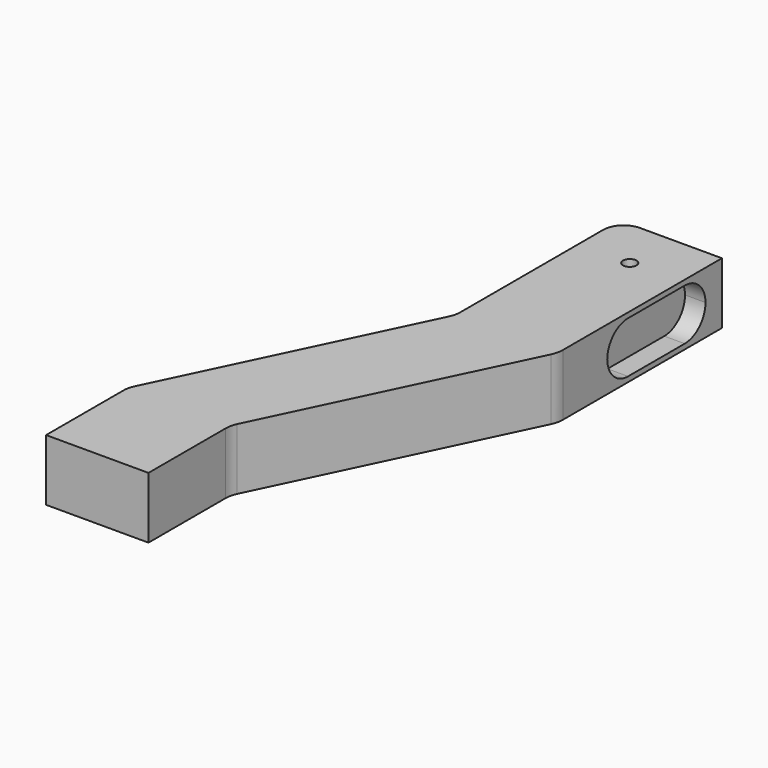
from build123d import *

# Parameters (mm, degrees)
F1_DEPTH    = 30
F2_W        = 60
F2_H        = 25
F3_DEPTH    = 10
F4_R        = 10
F5_R        = 3.2639
F6_DEPTH    = 30.001
F7_T1_DEPTH = 30
F7_T3_DEPTH = 10
F7_T5_DEPTH = 41.75
F7_T7_DEPTH = 44.4507439359


# Not quite as in the source:
# - a fillet or chamfer that OpenCascade refuses, or shapes differently, is made with other operations: its cross-section is extruded or revolved along the edge and cut away or added


with BuildPart() as f1:
    # F0 (on Top) → F1 (new body)
    with BuildSketch(Plane.XY):
        Polygon((-25, -100), (-25, -150), (25, -150), (25, -100), (85, 25), (85, 125), (35, 125), (35, 25), align=None)
    extrude(amount=F1_DEPTH)

    # F2 (on face) → F3 (cut)
    with BuildSketch(Plane.YZ.offset(85)):
        with Locations((85, 15)):
            Rectangle(F2_W, F2_H)
    extrude(amount=-F3_DEPTH, mode=Mode.SUBTRACT)

    # F4
    f4_edges = [f1.edges().sort_by_distance(p)[0] for p in [
        (35, 125, 15),
    ]]
    fillet(f4_edges, radius=F4_R)

    # F5 (on face) → F6 (cut, through all)
    with BuildSketch(Plane.XY.offset(30)):
        with Locations((60, 100)):
            Circle(F5_R)
    extrude(amount=-F6_DEPTH, mode=Mode.SUBTRACT)

    # F7: fillet of radius 12.7 on 8 edges, made by hand

    # F7_s2 → F7_t1 (join)
    with BuildSketch(Plane.XY):
        with BuildLine():
            ThreePointArc((26.2506571702, -97.3944642288), (25.3166108448, -100.0720513739), (25, -102.8901487872))
            Line((25, -102.8901487872), (25, -100))
            Line((25, -100), (26.2506571702, -97.3944642288))
        make_face()
        with BuildLine():
            ThreePointArc((35, 27.8901487872), (34.6833891552, 25.0720513739), (33.7493428298, 22.3944642288))
            Line((33.7493428298, 22.3944642288), (35, 25))
            Line((35, 25), (35, 27.8901487872))
        make_face()
    extrude(amount=F7_T1_DEPTH)

    # F7_s4 → F7_t3 (join)
    with BuildSketch(Plane.YZ.offset(75)):
        with BuildLine():
            ThreePointArc((102.3, 27.5), (111.2802561211, 23.7802561211), (115, 14.8))
            Line((115, 14.8), (115, 27.5))
            Line((115, 27.5), (102.3, 27.5))
        make_face()
        with BuildLine():
            ThreePointArc((115, 15.2), (111.2802561211, 6.2197438789), (102.3, 2.5))
            Line((102.3, 2.5), (115, 2.5))
            Line((115, 2.5), (115, 15.2))
        make_face()
    extrude(amount=F7_T3_DEPTH)

    # F7_s6 → F7_t5 (join)
    with BuildSketch(Plane.YZ.offset(43.25)):
        with BuildLine():
            ThreePointArc((67.7, 27.5), (58.7197438789, 23.7802561211), (55, 14.8))
            Line((55, 14.8), (55, 27.5))
            Line((55, 27.5), (67.7, 27.5))
        make_face()
        with BuildLine():
            ThreePointArc((67.7, 2.5), (58.7197438789, 6.2197438789), (55, 15.2))
            Line((55, 15.2), (55, 2.5))
            Line((55, 2.5), (67.7, 2.5))
        make_face()
    extrude(amount=F7_T5_DEPTH)

    # F7_s8 → F7_t7 (cut)
    with BuildSketch(Plane.XY.offset(-7.2253719679)):
        with BuildLine():
            ThreePointArc((85, 27.8901487872), (84.6833891552, 25.0720513739), (83.7493428298, 22.3944642288))
            Line((83.7493428298, 22.3944642288), (85, 25))
            Line((85, 25), (85, 27.8901487872))
        make_face()
        with BuildLine():
            ThreePointArc((-23.7493428298, -97.3944642288), (-24.6833891552, -100.0720513739), (-25, -102.8901487872))
            Line((-25, -102.8901487872), (-25, -100))
            Line((-25, -100), (-23.7493428298, -97.3944642288))
        make_face()
    extrude(amount=F7_T7_DEPTH, mode=Mode.SUBTRACT)


solid = f1.part
